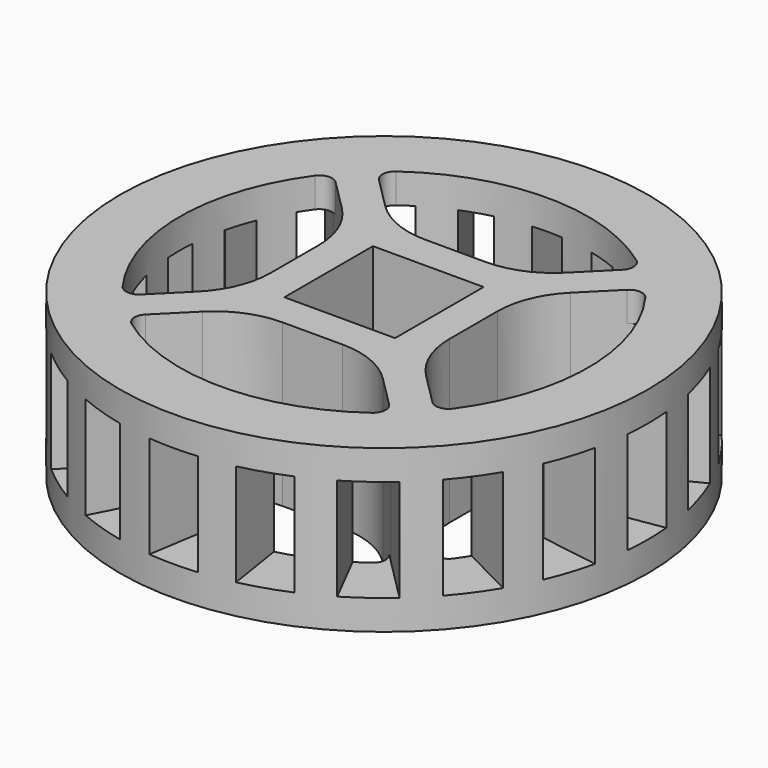
from build123d import *

# Parameters (mm, degrees)
F0_W             = 196.85
F0_H             = 120.65
F3_DEPTH         = 127
F3_COPIES_COUNT  = 4
F2_W             = 82.55
F2_H             = 82.55
F4_DEPTH         = 127
F5_DEPTH         = 38.1
F5_COPIES_COUNT  = 4
F5_COPIES_ANGLE  = 54
F5_COPIES1_COUNT = 4
F5_COPIES2_COUNT = 4
F5_COPIES2_ANGLE = 324
F6_T1_DEPTH      = 22.225
F6_T3_DEPTH      = 22.225


# Not quite as in the source:
# - a fillet or chamfer that OpenCascade refuses, or shapes differently, is made with other operations: its cross-section is extruded or revolved along the edge and cut away or added
# - a pattern or mirror of a feature is missing from the dataset's text; its kind, count and spacing are read off the source's solid


with BuildPart() as f1:
    # F0 (on Front) → F1 (revolve)
    with BuildSketch(Plane.XZ):
        with Locations((98.425, 0)):
            Rectangle(F0_W, F0_H)
    revolve(axis=Axis((0, 0, 0), (0, 0, 1)))

    # F2 (on Top) → F3 (cut, symmetric)
    with BuildSketch(Plane.XY):
        with BuildLine():
            Line((-85.2737193947, 67.3132071525), (-116.3685003566, 98.4079881145))
            ThreePointArc((-116.3685003566, 98.4079881145), (-123.2941899427, 89.5784724494), (-129.5514025719, 80.2632798461))
            ThreePointArc((-129.5514025719, 80.2632798461), (-151.9868585199, -11.2140464259), (-116.3685003566, -98.4079881145))
            Line((-116.3685003566, -98.4079881145), (-85.2737193947, -67.3132071525))
            ThreePointArc((-85.2737193947, -67.3132071525), (-71.5086496855, -46.7123245024), (-66.675, -22.4119265472))
            Line((-66.675, -22.4119265472), (-66.675, 22.4119265472))
            ThreePointArc((-66.675, 22.4119265472), (-71.5086496855, 46.7123245024), (-85.2737193947, 67.3132071525))
        make_face()
    f3 = extrude(amount=F3_DEPTH, both=True, mode=Mode.SUBTRACT)

    # F3_copies: F3 ×4 about axis
    f3_copies_axis = Axis((0, 0, 0), (0, 0, 1))
    for i in range(1, F3_COPIES_COUNT):
        add(f3.rotate(f3_copies_axis, i * 360 / F3_COPIES_COUNT), mode=Mode.SUBTRACT)

    # F2 (on Top) → F4 (cut, symmetric)
    with BuildSketch(Plane.XY):
        Rectangle(F2_W, F2_H)
    extrude(amount=F4_DEPTH, both=True, mode=Mode.SUBTRACT)

    # F2 (on Top) → F5 (cut, symmetric)
    with BuildSketch(Plane.XY):
        with BuildLine():
            ThreePointArc((-129.5514025719, 80.2632798461), (-123.2941899427, 89.5784724494), (-116.3685003566, 98.4079881145))
            Line((-116.3685003566, 98.4079881145), (-147.8842382454, 129.9237260033))
            ThreePointArc((-147.8842382454, 129.9237260033), (-159.2549953427, 115.7055269138), (-169.2635490548, 100.4976291331))
            Line((-169.2635490548, 100.4976291331), (-129.5514025719, 80.2632798461))
        make_face()
    f5 = extrude(amount=F5_DEPTH, both=True, mode=Mode.SUBTRACT)

    # F5_copies: F5 ×4 about axis
    f5_copies_axis = Axis((0, 0, 0), (0, 0, 1))
    for i in range(1, F5_COPIES_COUNT):
        add(f5.rotate(f5_copies_axis, i * F5_COPIES_ANGLE / (F5_COPIES_COUNT - 1)), mode=Mode.SUBTRACT)

    # F5_copies1: F5 ×4 about axis
    f5_copies1_axis = Axis((0, 0, 0), (0, 0, 1))
    for i in range(1, F5_COPIES1_COUNT):
        add(f5.rotate(f5_copies1_axis, i * 360 / F5_COPIES1_COUNT), mode=Mode.SUBTRACT)

    # F5_copies2: F5 ×4 about axis
    f5_copies2_axis = Axis((0, 0, 0), (0, 0, 1))
    for i in range(1, F5_COPIES2_COUNT):
        add(f5.rotate(f5_copies2_axis, i * F5_COPIES2_ANGLE / (F5_COPIES2_COUNT - 1)), mode=Mode.SUBTRACT)

    # F5_copies3: F5 across plane
    add(f5.mirror(Plane(origin=(0, 0, 0), x_dir=(-0.3090169944, 0.9510565163, 0), z_dir=(0.9510565163, 0.3090169944, 0))), mode=Mode.SUBTRACT)

    # F5_copies4: F5 across plane
    add(f5.mirror(Plane(origin=(0, 0, 0), x_dir=(-0.4539904997, 0.8910065242, 0), z_dir=(0.8910065242, 0.4539904997, 0))), mode=Mode.SUBTRACT)

    # F5_copies5: F5 across plane
    add(f5.mirror(Plane(origin=(0, 0, 0), x_dir=(0.7071067812, -0.7071067812, 0), z_dir=(0.7071067812, 0.7071067812, 0))), mode=Mode.SUBTRACT)

    # F5_copies6: F5 across plane
    add(f5.mirror(Plane(origin=(0, 0, 0), x_dir=(0, 0, 1), z_dir=(1, 0, 0))), mode=Mode.SUBTRACT)

    # F5_copies7: F5 across plane
    add(f5.mirror(Plane(origin=(0, 0, 0), x_dir=(0.156434465, 0.9876883406, 0), z_dir=(0.9876883406, -0.156434465, 0))), mode=Mode.SUBTRACT)

    # F5_copies8: F5 across plane
    add(f5.mirror(Plane(origin=(0, 0, 0), x_dir=(0.4539904997, 0.8910065242, 0), z_dir=(0.8910065242, -0.4539904997, 0))), mode=Mode.SUBTRACT)

    # F5_copies9: F5 across plane
    add(f5.mirror(Plane(origin=(0, 0, 0), x_dir=(-0.7071067812, -0.7071067812, 0), z_dir=(0.7071067812, -0.7071067812, 0))), mode=Mode.SUBTRACT)

    # F5_copies10: F5 across plane
    add(f5.mirror(Plane(origin=(0, 0, 0), x_dir=(-0.8090169944, -0.5877852523, 0), z_dir=(0.5877852523, -0.8090169944, 0))), mode=Mode.SUBTRACT)

    # F5_copies11: F5 across plane
    add(f5.mirror(Plane(origin=(0, 0, 0), x_dir=(-0.8910065242, -0.4539904997, 0), z_dir=(0.4539904997, -0.8910065242, 0))), mode=Mode.SUBTRACT)

    # F5_copies12: F5 across plane
    add(f5.mirror(Plane(origin=(0, 0, 0), x_dir=(0, 0, -1), z_dir=(0, -1, 0))), mode=Mode.SUBTRACT)

    # F6: fillet of radius 9.525 on 16 edges, made by hand

    # F6_s2 → F6_t1 (join)
    with BuildSketch(Plane.XY.offset(38.1)):
        with BuildLine():
            ThreePointArc((-123.2144339849, -89.6881444662), (-116.2566300522, -93.578604586), (-108.77833977, -90.8178275279))
            Line((-108.77833977, -90.8178275279), (-116.3685003566, -98.4079881145))
            ThreePointArc((-116.3685003566, -98.4079881145), (-119.8707826171, -94.1103367052), (-123.2144339849, -89.6881444662))
        make_face()
        with BuildLine():
            ThreePointArc((-108.77833977, 90.8178275279), (-116.2566300522, 93.578604586), (-123.2144339849, 89.6881444662))
            ThreePointArc((-123.2144339849, 89.6881444662), (-119.8707826171, 94.1103367052), (-116.3685003566, 98.4079881145))
            Line((-116.3685003566, 98.4079881145), (-108.77833977, 90.8178275279))
        make_face()
        with BuildLine():
            ThreePointArc((-90.8178275279, -108.77833977), (-93.578604586, -116.2566300522), (-89.6881444662, -123.2144339849))
            ThreePointArc((-89.6881444662, -123.2144339849), (-94.1103367052, -119.8707826171), (-98.4079881145, -116.3685003566))
            Line((-98.4079881145, -116.3685003566), (-90.8178275279, -108.77833977))
        make_face()
        with BuildLine():
            ThreePointArc((89.6881444662, -123.2144339849), (93.578604586, -116.2566300522), (90.8178275279, -108.77833977))
            Line((90.8178275279, -108.77833977), (98.4079881145, -116.3685003566))
            ThreePointArc((98.4079881145, -116.3685003566), (94.1103367052, -119.8707826171), (89.6881444662, -123.2144339849))
        make_face()
        with BuildLine():
            ThreePointArc((108.77833977, -90.8178275279), (116.2566300522, -93.578604586), (123.2144339849, -89.6881444662))
            ThreePointArc((123.2144339849, -89.6881444662), (119.8707826171, -94.1103367052), (116.3685003566, -98.4079881145))
            Line((116.3685003566, -98.4079881145), (108.77833977, -90.8178275279))
        make_face()
        with BuildLine():
            ThreePointArc((123.2144339849, 89.6881444662), (116.2566300522, 93.578604586), (108.77833977, 90.8178275279))
            Line((108.77833977, 90.8178275279), (116.3685003566, 98.4079881145))
            ThreePointArc((116.3685003566, 98.4079881145), (119.8707826171, 94.1103367052), (123.2144339849, 89.6881444662))
        make_face()
        with BuildLine():
            ThreePointArc((90.8178275279, 108.77833977), (93.578604586, 116.2566300522), (89.6881444662, 123.2144339849))
            ThreePointArc((89.6881444662, 123.2144339849), (94.1103367052, 119.8707826171), (98.4079881145, 116.3685003566))
            Line((98.4079881145, 116.3685003566), (90.8178275279, 108.77833977))
        make_face()
        with BuildLine():
            ThreePointArc((-89.6881444662, 123.2144339849), (-93.578604586, 116.2566300522), (-90.8178275279, 108.77833977))
            Line((-90.8178275279, 108.77833977), (-98.4079881145, 116.3685003566))
            ThreePointArc((-98.4079881145, 116.3685003566), (-94.1103367052, 119.8707826171), (-89.6881444662, 123.2144339849))
        make_face()
    extrude(amount=F6_T1_DEPTH)

    # F6_s4 → F6_t3 (join)
    with BuildSketch(Plane.XY.offset(-60.325)):
        with BuildLine():
            ThreePointArc((-123.2144339849, -89.6881444662), (-116.2566300522, -93.578604586), (-108.77833977, -90.8178275279))
            Line((-108.77833977, -90.8178275279), (-116.3685003566, -98.4079881145))
            ThreePointArc((-116.3685003566, -98.4079881145), (-119.8707826171, -94.1103367052), (-123.2144339849, -89.6881444662))
        make_face()
        with BuildLine():
            ThreePointArc((-108.77833977, 90.8178275279), (-116.2566300522, 93.578604586), (-123.2144339849, 89.6881444662))
            ThreePointArc((-123.2144339849, 89.6881444662), (-119.8707826171, 94.1103367052), (-116.3685003566, 98.4079881145))
            Line((-116.3685003566, 98.4079881145), (-108.77833977, 90.8178275279))
        make_face()
        with BuildLine():
            ThreePointArc((-90.8178275279, -108.77833977), (-93.578604586, -116.2566300522), (-89.6881444662, -123.2144339849))
            ThreePointArc((-89.6881444662, -123.2144339849), (-94.1103367052, -119.8707826171), (-98.4079881145, -116.3685003566))
            Line((-98.4079881145, -116.3685003566), (-90.8178275279, -108.77833977))
        make_face()
        with BuildLine():
            ThreePointArc((89.6881444662, -123.2144339849), (93.578604586, -116.2566300522), (90.8178275279, -108.77833977))
            Line((90.8178275279, -108.77833977), (98.4079881145, -116.3685003566))
            ThreePointArc((98.4079881145, -116.3685003566), (94.1103367052, -119.8707826171), (89.6881444662, -123.2144339849))
        make_face()
        with BuildLine():
            ThreePointArc((108.77833977, -90.8178275279), (116.2566300522, -93.578604586), (123.2144339849, -89.6881444662))
            ThreePointArc((123.2144339849, -89.6881444662), (119.8707826171, -94.1103367052), (116.3685003566, -98.4079881145))
            Line((116.3685003566, -98.4079881145), (108.77833977, -90.8178275279))
        make_face()
        with BuildLine():
            ThreePointArc((123.2144339849, 89.6881444662), (116.2566300522, 93.578604586), (108.77833977, 90.8178275279))
            Line((108.77833977, 90.8178275279), (116.3685003566, 98.4079881145))
            ThreePointArc((116.3685003566, 98.4079881145), (119.8707826171, 94.1103367052), (123.2144339849, 89.6881444662))
        make_face()
        with BuildLine():
            ThreePointArc((90.8178275279, 108.77833977), (93.578604586, 116.2566300522), (89.6881444662, 123.2144339849))
            ThreePointArc((89.6881444662, 123.2144339849), (94.1103367052, 119.8707826171), (98.4079881145, 116.3685003566))
            Line((98.4079881145, 116.3685003566), (90.8178275279, 108.77833977))
        make_face()
        with BuildLine():
            ThreePointArc((-89.6881444662, 123.2144339849), (-93.578604586, 116.2566300522), (-90.8178275279, 108.77833977))
            Line((-90.8178275279, 108.77833977), (-98.4079881145, 116.3685003566))
            ThreePointArc((-98.4079881145, 116.3685003566), (-94.1103367052, 119.8707826171), (-89.6881444662, 123.2144339849))
        make_face()
    extrude(amount=F6_T3_DEPTH)


solid = f1.part
